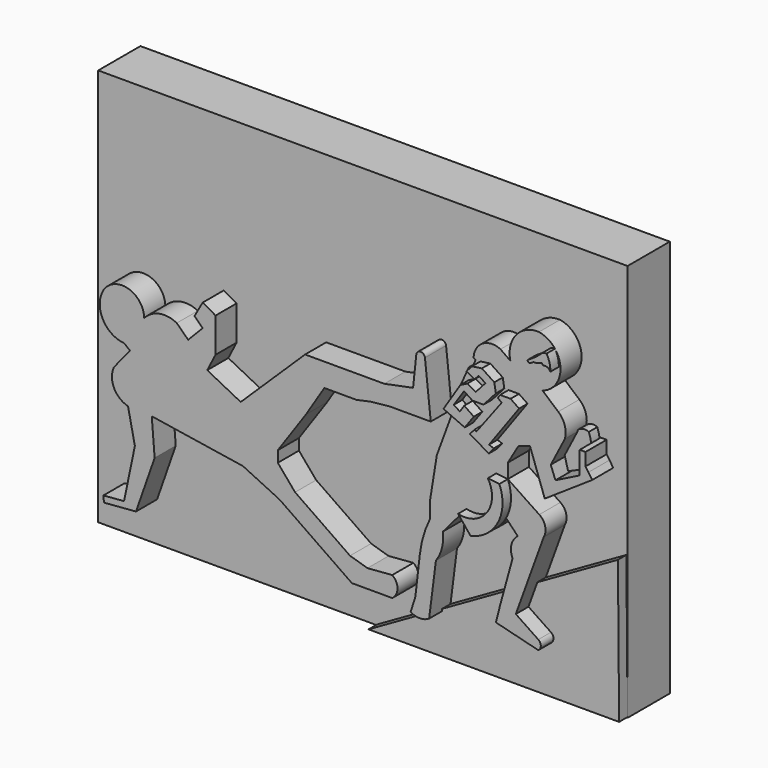
from build123d import *

# Parameters (mm, degrees)
F0_W     = 127.4373829365
F0_H     = 95.7600027323
F1_DEPTH = 12.7
F4_DEPTH = 2.54
F5_DEPTH = 6.35
F7_DEPTH = 6.35
F9_DEPTH = 2.54


with BuildPart() as f1:
    # F0 (on Front) → F1 (new body)
    with BuildSketch(Plane.XZ):
        with Locations((-24.3238061666, -2.5199986994)):
            Rectangle(F0_W, F0_H)
    extrude(amount=F1_DEPTH)

    # F6 (on face) → F7 (join)
    with BuildSketch(Plane.XZ.offset(12.7)):
        with BuildLine():
            Line((-6.6146305762, -37.1381999661), (-7.7518131584, -40.7059751451))
            ThreePointArc((-7.7518131584, -40.7059751451), (-5.5234554805, -41.3317383256), (-3.302536672, -40.6800657511))
            Line((-3.302536672, -40.6800657511), (-1.6684934963, -27.850324288))
            ThreePointArc((-1.6684934963, -27.850324288), (-0.1977433329, -24.6675530857), (0, -21.1669765413))
            Line((0, -21.1669765413), (5.7072923519, -14.4983688369))
            Line((5.7072923519, -14.4983688369), (8.6832400411, -18.1926488876))
            ThreePointArc((8.6832400411, -18.1926488876), (12.5118324121, -16.5297212642), (15.3534682468, -13.4721808136))
            Line((15.3534682468, -13.4721808136), (18.0215593427, -16.2428896874))
            ThreePointArc((18.0215593427, -16.2428896874), (16.507748126, -18.5928186122), (16.7901329696, -21.373834461))
            Line((16.7901329696, -21.373834461), (13.7659466469, -32.3677430681))
            Line((13.7659466469, -32.3677430681), (12.78799586, -36.2535752356))
            Line((12.78799586, -36.2535752356), (22.9817442596, -38.8190448284))
            ThreePointArc((22.9817442596, -38.8190448284), (23.5808314048, -37.6928821206), (22.9817442596, -36.5667194128))
            Line((22.9817442596, -36.5667194128), (17.5697784871, -32.9195261002))
            Line((17.5697784871, -32.9195261002), (24.2759082466, -14.4482571632))
            ThreePointArc((24.2759082466, -14.4482571632), (24.6242949781, -12.0173546169), (23.2220198959, -10.0013474002))
            Line((23.2220198959, -10.0013474002), (15.6425405294, -4.9483603798))
            Line((15.6425405294, -4.9483603798), (15.6425405294, -1.4699846506))
            Line((15.6425405294, -1.4699846506), (18.1591961987, 2.8296455063))
            Line((18.1591961987, 2.8296455063), (20.9683617805, 3.8287823554))
            Line((20.9683617805, 3.8287823554), (24.5338678045, -6.1959673201))
            Line((24.5338678045, -6.1959673201), (35.9428529965, 1.4582823496))
            Line((35.9428529965, 1.4582823496), (35.0417229934, 2.8014550061))
            Line((35.0417229934, 2.8014550061), (34.3524925411, 3.8287823554))
            Line((34.3524925411, 3.8287823554), (34.3524925411, 6.8964906968))
            Line((34.3524925411, 6.8964906968), (32.9580791295, 6.8964906968))
            Line((32.9580791295, 6.8964906968), (32.9580791295, 1.4582823496))
            Line((32.9580791295, 1.4582823496), (27.1015502512, -1.4699846506))
            Line((27.1015502512, -1.4699846506), (25.9860176593, 1.4582823496))
            Line((25.9860176593, 1.4582823496), (29.3974466622, 8.0836592242))
            ThreePointArc((29.3974466622, 8.0836592242), (29.3375005478, 10.919586761), (27.7805011719, 13.2906269282))
            Line((27.7805011719, 13.2906269282), (23.9999741316, 16.5386870503))
            ThreePointArc((23.9999741316, 16.5386870503), (28.3165834088, 22.9416425188), (23.1480244547, 28.6789722741))
            ThreePointArc((23.1480244547, 28.6789722741), (17.613067936, 26.2273412386), (16.2518583238, 20.3287526965))
            Line((16.2518583238, 20.3287526965), (13.8825792819, 22.0045838505))
            ThreePointArc((13.8825792819, 22.0045838505), (9.550247135, 21.7852106262), (7.4084724309, 18.0129397505))
            Line((7.4084724309, 18.0129397505), (7.8945502721, 17.7959588019))
            Line((7.8945502721, 17.7959588019), (6.84406026, 15.4426650196))
            Line((6.84406026, 15.4426650196), (6.2546562403, 15.7057698816))
            Line((6.2546562403, 15.7057698816), (1.5152784367, 5.0886786297))
            Line((1.5152784367, 5.0886786297), (2.3157484829, 4.7944039106))
            Line((2.3157484829, 4.7944039106), (-1.451083459, -5.4519269615))
            Line((-1.451083459, -5.4519269615), (-3.0324391555, -15.2601888403))
            Line((-3.0324391555, -15.2601888403), (-3.0324391555, -19.3585418165))
            ThreePointArc((-3.0324391555, -19.3585418165), (-4.659697335, -23.4949679023), (-5.5478756392, -27.850324288))
            Line((-5.5478756392, -27.850324288), (-6.6146305762, -37.1381999661))
        make_face()
    extrude(amount=F7_DEPTH)


with BuildPart() as f4:
    # F3 (on face) → F4 (new body)
    with BuildSketch(Plane.XZ.offset(12.7)):
        Polygon((39.3851324916, -50.2357855439), (39.1019172966, -15.9671995789), (-20.9389086813, -50.2357855439), align=None)
    extrude(amount=F4_DEPTH)


with BuildPart() as f4b:
    # F3 (on face) → F4, piece 2 (new body)
    with BuildSketch(Plane.XZ.offset(12.7)):
        with BuildLine():
            ThreePointArc((31.5112024546, 0.8082241402), (32.7042745556, 4.7667185798), (32.0980511606, 8.8564120233))
            ThreePointArc((32.0980511606, 8.8564120233), (30.4667649294, 8.9933431924), (29.121896252, 8.0599766225))
            Line((29.121896252, 8.0599766225), (26.2714978307, 2.0657528657))
            Line((26.2714978307, 2.0657528657), (27.109850198, -1.0780703742))
            Line((27.109850198, -1.0780703742), (31.5112024546, 0.8082241402))
        make_face()
    extrude(amount=F4_DEPTH)


with BuildPart() as f5:
    # F2 (on face) → F5 (new body)
    with BuildSketch(Plane.XZ.offset(12.7)):
        with BuildLine():
            Line((-69.3795382977, -28.1010381877), (-70.071734488, -19.498039037))
            Line((-70.071734488, -19.498039037), (-48.1178425252, -22.924637422))
            Line((-48.1178425252, -22.924637422), (-39.2935272157, -27.1558395766))
            Line((-39.2935272157, -27.1558395766), (-27.6997792235, -35.1822776493))
            Line((-27.6997792235, -35.1822776493), (-21.8916106969, -39.2033159733))
            Line((-21.8916106969, -39.2033159733), (-12.1742398351, -39.2033159733))
            ThreePointArc((-12.1742398351, -39.2033159733), (-10.9098976308, -36.7649858596), (-12.1742398351, -34.326655746))
            Line((-12.1742398351, -34.326655746), (-18.1467756629, -34.8072052002))
            Line((-18.1467756629, -34.8072052002), (-22.343594153, -33.5424220646))
            Line((-22.343594153, -33.5424220646), (-35.5684012175, -24.3867896497))
            Line((-35.5684012175, -24.3867896497), (-39.7254787385, -19.498039037))
            Line((-39.7254787385, -19.498039037), (-39.7254787385, -16.8267451227))
            Line((-39.7254787385, -16.8267451227), (-32.9544059932, -7.0463032462))
            Line((-32.9544059932, -7.0463032462), (-28.5239480436, 0))
            Line((-28.5239480436, 0), (-20.7618977875, 0))
            Line((-20.7618977875, 0), (-17.4428516504, 0.716215347))
            Line((-17.4428516504, 0.716215347), (-12.8509569913, 1.2057434514))
            Line((-12.8509569913, 1.2057434514), (-2.9095075055, 1.2057434514))
            Line((-2.9095075055, 1.2057434514), (-4.3040225282, 14.2866391689))
            ThreePointArc((-4.3040225282, 14.2866391689), (-5.3458241746, 15.2232808086), (-6.3876258209, 14.2866391689))
            Line((-6.3876258209, 14.2866391689), (-7.1662967093, 6.9825137034))
            Line((-7.1662967093, 6.9825137034), (-14.0896616504, 5.5874628015))
            Line((-14.0896616504, 5.5874628015), (-33.1655144691, 5.5874628015))
            Line((-33.1655144691, 5.5874628015), (-48.6597352362, -9.5206420708))
            Line((-48.6597352362, -9.5206420708), (-56.7218251526, -5.3977933712))
            Line((-56.7218251526, -5.3977933712), (-54.7203769951, -1.4840298099))
            Line((-54.7203769951, -1.4840298099), (-54.7203769951, 3.1556141155))
            Line((-54.7203769951, 3.1556141155), (-54.7203769951, 6.8316494449))
            Line((-54.7203769951, 6.8316494449), (-57.8110309296, 8.5799321532))
            Line((-57.8110309296, 8.5799321532), (-59.793189331, 5.0758274493))
            Line((-59.793189331, 5.0758274493), (-57.8110309296, 3.1556141155))
            Line((-57.8110309296, 3.1556141155), (-61.3084643152, -0.4546446233))
            Line((-61.3084643152, -0.4546446233), (-64.055425934, 2.2064708173))
            ThreePointArc((-64.055425934, 2.2064708173), (-68.221909624, 2.831049614), (-71.8791241567, 0.7395269931))
            ThreePointArc((-71.8791241567, 0.7395269931), (-75.7417583856, 5.719417786), (-81.6528702895, 3.5335514694))
            ThreePointArc((-81.6528702895, 3.5335514694), (-81.8856925895, -2.709846974), (-76.6969750444, -6.18999648))
            Line((-76.6969750444, -6.18999648), (-75.3276497126, -7.2959894314))
            Line((-75.3276497126, -7.2959894314), (-79.1822299361, -12.068329379))
            ThreePointArc((-79.1822299361, -12.068329379), (-79.1680295911, -16.4462375496), (-75.7865309715, -19.2268397659))
            Line((-75.7865309715, -19.2268397659), (-74.1345658898, -27.1195564419))
            Line((-74.1345658898, -27.1195564419), (-76.7466444413, -39.6645964929))
            Line((-76.7466444413, -39.6645964929), (-81.7051546826, -40.0635575806))
            Line((-81.7051546826, -40.0635575806), (-81.5855221327, -41.5504174326))
            Line((-81.5855221327, -41.5504174326), (-73.8695263863, -40.9295894206))
            Line((-73.8695263863, -40.9295894206), (-69.3795382977, -28.1010381877))
        make_face()
    extrude(amount=F5_DEPTH)


with BuildPart() as f9:
    # F8 (on face) → F9 (new body)
    with BuildSketch(Plane.XZ.offset(19.05)):
        with BuildLine():
            Line((15.6425405294, -4.9483603798), (12.862472795, -4.6370709315))
            ThreePointArc((12.862472795, -4.6370709315), (12.6280677838, -11.9934749587), (5.7072923519, -14.4983688369))
            Line((5.7072923519, -14.4983688369), (8.6832400411, -18.1926488876))
            ThreePointArc((8.6832400411, -18.1926488876), (15.2999989561, -13.2189194876), (15.6425405294, -4.9483603798))
        make_face()
    extrude(amount=F9_DEPTH)


with BuildPart() as f9b:
    # F8 (on face) → F9, piece 2 (new body)
    with BuildSketch(Plane.XZ.offset(19.05)):
        Polygon((7.3064081371, 4.3127438985), (9.4912303612, 7.3262914084), (7.1804024406, 8.894868966), (6.1290945258, 7.3056530198), (4.675580153, 8.2671907944), (7.1201149447, 11.9624865472), (9.1521320865, 10.6182540601), (11.8264881668, 10.6182540601), (14.8089015856, 13.9854960144), (14.4205187694, 16.1995759515), (11.4278439432, 18.1793086231), (9.037706329, 17.8403760046), (7.7541945502, 16.3912493736), (9.6918641893, 15.3121929616), (10.6475995854, 16.3912493736), (12.2787617147, 15.3121929616), (9.9432626739, 12.6753384247), (7.9091172665, 13.8054192066), (6.2546562403, 12.9766939208), (2.1886910356, 6.5972485957), align=None)
    extrude(amount=F9_DEPTH)


with BuildPart() as f9c:
    # F8 (on face) → F9, piece 3 (new body)
    with BuildSketch(Plane.XZ.offset(19.05)):
        Polygon((15.2530662198, 13.1327583484), (16.226509586, 12.488800101), (10.096295092, 4.328647619), (9.7036249936, 4.6722339466), (8.5271028802, 3.3276372124), (13.1071358919, 0.6804620498), (14.2836580053, 2.1511148661), (13.1491543725, 2.5713017676), (20.3882604837, 12.5802671537), (18.330251798, 13.9818962362), (15.814793142, 13.9818962362), align=None)
    extrude(amount=F9_DEPTH)


with BuildPart() as f9d:
    # F8 (on face) → F9, piece 4 (new body)
    with BuildSketch(Plane.XZ.offset(19.05)):
        with BuildLine():
            ThreePointArc((25.4105795175, 25.6545562297), (23.9945449148, 24.5392157595), (22.4735308439, 23.5719233751))
            ThreePointArc((22.4735308439, 23.5719233751), (22.6322049019, 23.1166423149), (23.1143422425, 23.1180153787))
            Line((23.1143422425, 23.1180153787), (23.8886550069, 23.5719233751))
            Line((23.8886550069, 23.5719233751), (24.4760643691, 23.5719233751))
            Line((24.4760643691, 23.5719233751), (25.8644875139, 23.9724293351))
            Line((25.8644875139, 23.9724293351), (26.1314902455, 23.5719233751))
            ThreePointArc((26.1314902455, 23.5719233751), (27.1703281511, 23.5435806354), (27.9204212129, 22.8243116289))
            ThreePointArc((27.9204212129, 22.8243116289), (27.7128438446, 24.6661490518), (26.9939674665, 26.3745606558))
            ThreePointArc((26.9939674665, 26.3745606558), (26.1101959802, 26.2170494514), (25.4105795175, 25.6545562297))
        make_face()
    extrude(amount=F9_DEPTH)


solid = Compound([f1.part, f4.part, f4b.part, f5.part, f9.part, f9b.part, f9c.part, f9d.part])
